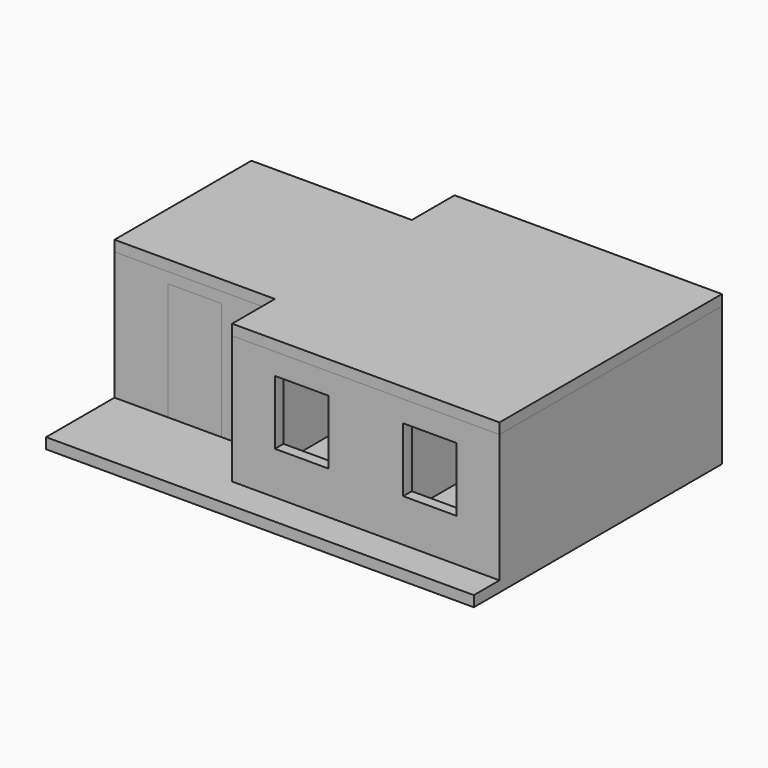
from build123d import *

# Parameters (mm, degrees)
F0_W      = 1828.8
F0_H      = 304.8
F1_DEPTH  = 3657.6
F0_W_2    = 1524
F0_W_3    = 1219.2
F0_W_4    = 914.4
F0_W_5    = 609.6
F2_W      = 12192
F2_H      = 7924.8
F2_H_2    = 914.4
F3_DEPTH  = 304.8
F4_W      = 2133.6
F4_H      = 304.8
F4_W_2    = 1524
F5_DEPTH  = 1219.2
F7_W      = 2133.6
F7_H      = 304.8
F7_W_2    = 1524
F8_DEPTH  = 609.6
F11_DEPTH = 304.8
F13_W     = 1524
F13_H     = 30.48
F14_DEPTH = 3352.8
F13_W_2   = 914.4
F15_W     = 1524
F15_H     = 304.8
F16_DEPTH = 1219.2
F17_W     = 457.2
F17_H     = 2286
F18_DEPTH = 914.4
F19_W     = 1066.8
F19_H     = 609.6
F19_W_2   = 609.6
F19_H_2   = 2133.6
F20_DEPTH = 609.6
F21_W     = 1066.8
F21_H     = 152.4
F21_W_2   = 152.4
F21_H_2   = 2133.6
F22_DEPTH = 609.6
F23_R     = 152.4
F24_DEPTH = 457.2
F24_TAPER = 10
F25_R     = 457.2
F26_DEPTH = 30.48
F27_W     = 914.4
F27_H     = 304.8
F27_W_2   = 1524
F28_DEPTH = 304.8
F29_W     = 1524
F29_H     = 30.48
F30_DEPTH = 1828.8
F31_W     = 2133.6
F31_H     = 74.5021455099
F32_DEPTH = 1828.8


with BuildPart() as f1:
    # F0 (on Top) → F1 (new body)
    with BuildSketch(Plane.XY):
        Polygon((-1524, -1337.5231116007), (-1524, -1642.3231116007), (0, -1642.3231116007), (0, -1337.5231116007), (-1219.2, -1337.5231116007), align=None)
        Polygon((-1524, 3234.4768883993), (-1524, -1337.5231116007), (-1219.2, -1337.5231116007), (-1219.2, 2929.6768883993), (-1219.2, 3234.4768883993), align=None)
        with Locations((-304.8, 3082.0768883993)):
            Rectangle(F0_W, F0_H)
    extrude(amount=F1_DEPTH)



with BuildPart() as f1b:
    # F0 (on Top) → F1, piece 2 (new body)
    with BuildSketch(Plane.XY):
        with Locations((2286, -1489.9231116007)):
            Rectangle(F0_W_2, F0_H)
        Polygon((3048, 186.4768883993), (3048, -1337.5231116007), (3048, -1642.3231116007), (3048, -3166.3231116007), (3352.8, -3166.3231116007), (3352.8, -2861.5231116007), (3352.8, -118.3231116007), (3352.8, 186.4768883993), align=None)
        with Locations((3962.4, 34.0768883993)):
            Rectangle(F0_W_3, F0_H)
        with Locations((3810, -3013.9231116007)):
            Rectangle(F0_W_4, F0_H)
    extrude(amount=F1_DEPTH)


with BuildPart() as f1c:
    # F0 (on Top) → F1, piece 3 (new body)
    with BuildSketch(Plane.XY):
        with Locations((2286, 3082.0768883993)):
            Rectangle(F0_W_2, F0_H)
        Polygon((3048, 4758.4768883993), (3048, 3234.4768883993), (3048, 2929.6768883993), (3048, 1405.6768883993), (3352.8, 1405.6768883993), (3352.8, 1710.4768883993), (3352.8, 4453.6768883993), (3352.8, 4758.4768883993), align=None)
        with Locations((3657.6, 4606.0768883993)):
            Rectangle(F0_W_5, F0_H)
        with Locations((3962.4, 1558.0768883993)):
            Rectangle(F0_W_3, F0_H)
    extrude(amount=F1_DEPTH)


with BuildPart() as f1d:
    # F0 (on Top) → F1, piece 4 (new body)
    with BuildSketch(Plane.XY):
        with Locations((6096, 1558.0768883993)):
            Rectangle(F0_W_3, F0_H)
        Polygon((6705.6, 4453.6768883993), (6705.6, 1710.4768883993), (6705.6, 1405.6768883993), (7010.4, 1405.6768883993), (7010.4, 1710.4768883993), (7010.4, 4453.6768883993), (7010.4, 4758.4768883993), (6705.6, 4758.4768883993), align=None)
        with Locations((6400.8, 4606.0768883993)):
            Rectangle(F0_W_5, F0_H)
        with Locations((7620, 1558.0768883993)):
            Rectangle(F0_W_3, F0_H)
        with Locations((7467.6, 4606.0768883993)):
            Rectangle(F0_W_4, F0_H)
    extrude(amount=F1_DEPTH)


with BuildPart() as f1e:
    # F0 (on Top) → F1, piece 5 (new body)
    with BuildSketch(Plane.XY):
        with Locations((6096, 34.0768883993)):
            Rectangle(F0_W_3, F0_H)
        Polygon((7010.4, 186.4768883993), (6705.6, 186.4768883993), (6705.6, -118.3231116007), (6705.6, -2861.5231116007), (6705.6, -3166.3231116007), (7010.4, -3166.3231116007), (7010.4, -2861.5231116007), (7010.4, -118.3231116007), align=None)
        with Locations((7620, 34.0768883993)):
            Rectangle(F0_W_3, F0_H)
        with Locations((6248.4, -3013.9231116007)):
            Rectangle(F0_W_4, F0_H)
        with Locations((7467.6, -3013.9231116007)):
            Rectangle(F0_W_4, F0_H)
    extrude(amount=F1_DEPTH)


with BuildPart() as f1f:
    # F0 (on Top) → F1, piece 6 (new body)
    with BuildSketch(Plane.XY):
        with Locations((9906, 4606.0768883993)):
            Rectangle(F0_W_4, F0_H)
        Polygon((10668, 4758.4768883993), (10363.2, 4758.4768883993), (10363.2, 4453.6768883993), (10363.2, 1710.4768883993), (10363.2, 1405.6768883993), (10668, 1405.6768883993), align=None)
        with Locations((9753.6, 1558.0768883993)):
            Rectangle(F0_W_3, F0_H)
        Polygon((10668, -3166.3231116007), (10668, 1405.6768883993), (10363.2, 1405.6768883993), (10363.2, 186.4768883993), (10363.2, -118.3231116007), (10363.2, -2861.5231116007), (10363.2, -3166.3231116007), align=None)
        with Locations((9753.6, 34.0768883993)):
            Rectangle(F0_W_3, F0_H)
        with Locations((9906, -3013.9231116007)):
            Rectangle(F0_W_4, F0_H)
    extrude(amount=F1_DEPTH)


with BuildPart() as f1_1:
    add(f1.part)

    add(f1b.part)  # F3 merges F1b

    add(f1c.part)  # F3 merges F1c

    add(f1d.part)  # F3 merges F1d

    add(f1e.part)  # F3 merges F1e

    add(f1f.part)  # F3 merges F1f
    # F2 (on Top) → F3 (join)
    with BuildSketch(Plane.XY):
        with Locations((4572, 796.0768883993)):
            Rectangle(F2_W, F2_H)
        with Locations((4572, -3623.5231116007)):
            Rectangle(F2_W, F2_H_2)
    extrude(amount=-F3_DEPTH)

    # F4 (on Top) → F5 (join)
    with BuildSketch(Plane.XY):
        with Locations((5029.2, 4606.0768883993)):
            Rectangle(F4_W, F4_H)
        with Locations((8686.8, -3013.9231116007)):
            Rectangle(F4_W_2, F4_H)
        with Locations((5029.2, -3013.9231116007)):
            Rectangle(F4_W_2, F4_H)
    extrude(amount=F5_DEPTH)

    # F7 (on offset) → F8 (join)
    with BuildSketch(Plane.XY.offset(3048)):
        with Locations((5029.2, 4606.0768883993)):
            Rectangle(F7_W, F7_H)
        with Locations((8686.8, 4606.0768883993)):
            Rectangle(F7_W_2, F7_H)
        with Locations((8686.8, -3013.9231116007)):
            Rectangle(F7_W_2, F7_H)
        with Locations((5029.2, -3013.9231116007)):
            Rectangle(F7_W_2, F7_H)
    extrude(amount=F8_DEPTH)

    # F12: union 

    # F15 (on Top) → F16 (join)
    with BuildSketch(Plane.XY):
        with Locations((8686.8, 4606.0768883993)):
            Rectangle(F15_W, F15_H)
    extrude(amount=F16_DEPTH)

    # F17 (on Top) → F18 (join)
    with BuildSketch(Plane.XY):
        Polygon((6705.6, 4453.6768883993), (3352.8, 4453.6768883993), (3352.8, 3996.4768883993), (6248.4, 3996.4768883993), (6705.6, 3996.4768883993), align=None)
        with Locations((6477, 2853.4768883993)):
            Rectangle(F17_W, F17_H)
    extrude(amount=F18_DEPTH)

    # F19 (on Top) → F20 (join)
    with BuildSketch(Plane.XY):
        with Locations((76.2, 2472.4768883993)):
            Rectangle(F19_W, F19_H)
        with Locations((-762, 643.6768883993)):
            Rectangle(F19_W_2, F19_H_2)
    extrude(amount=F20_DEPTH)

    # F21 (on face) → F22 (join)
    with BuildSketch(Plane.XY.offset(609.6)):
        with Locations((76.2, 2701.0768883993)):
            Rectangle(F21_W, F21_H)
        with Locations((-990.6, 643.6768883993)):
            Rectangle(F21_W_2, F21_H_2)
    extrude(amount=F22_DEPTH)

    # F23 (on Top) → F24 (join)
    with BuildSketch(Plane.XY):
        with Locations((527.5880694389, 676.9324541092)):
            Circle(F23_R)
    extrude(amount=F24_DEPTH, taper=F24_TAPER)

    # F25 (on face) → F26 (join)
    with BuildSketch(Plane.XY.offset(457.2)):
        with Locations((527.5880694389, 676.9324541092)):
            Circle(F25_R)
    extrude(amount=F26_DEPTH)

    # F27 (on face) → F28 (join)
    with BuildSketch(Plane.XY.offset(3352.8)):
        with Locations((1066.8, 3082.0768883993)):
            Rectangle(F27_W, F27_H)
        with Locations((762, -1489.9231116007)):
            Rectangle(F27_W_2, F27_H)
    extrude(amount=F28_DEPTH)


with BuildPart() as f11:
    # F10 (on offset) → F11 (new body)
    with BuildSketch(Plane.XY.offset(3657.6)):
        Polygon((3048, 3234.4768883993), (-1524, 3234.4768883993), (-1524, -1642.3231116007), (3048, -1642.3231116007), (3048, -3166.3231116007), (10668, -3166.3231116007), (10668, 4758.4768883993), (3048, 4758.4768883993), align=None)
    extrude(amount=F11_DEPTH)


with BuildPart() as f14:
    # F13 (on Top) → F14 (new body)
    with BuildSketch(Plane.XY):
        with Locations((762, -1627.0831116007)):
            Rectangle(F13_W, F13_H)
    extrude(amount=F14_DEPTH)


with BuildPart() as f14b:
    # F13 (on Top) → F14, piece 2 (new body)
    with BuildSketch(Plane.XY):
        with Locations((1066.8, 3219.2368883993)):
            Rectangle(F13_W_2, F13_H)
    extrude(amount=F14_DEPTH)


with BuildPart() as f30:
    # F29 (on face) → F30 (new body)
    with BuildSketch(Plane.XY.offset(1219.2)):
        with Locations((8686.8, 4743.2368883993)):
            Rectangle(F29_W, F29_H)
    extrude(amount=F30_DEPTH)


with BuildPart() as f32:
    # F31 (on face) → F32 (new body)
    with BuildSketch(Plane.XY.offset(1219.2)):
        with Locations((5029.2, 4721.2258156443)):
            Rectangle(F31_W, F31_H)
    extrude(amount=F32_DEPTH)


solid = Compound([f1_1.part, f11.part, f14.part, f14b.part, f30.part, f32.part])
